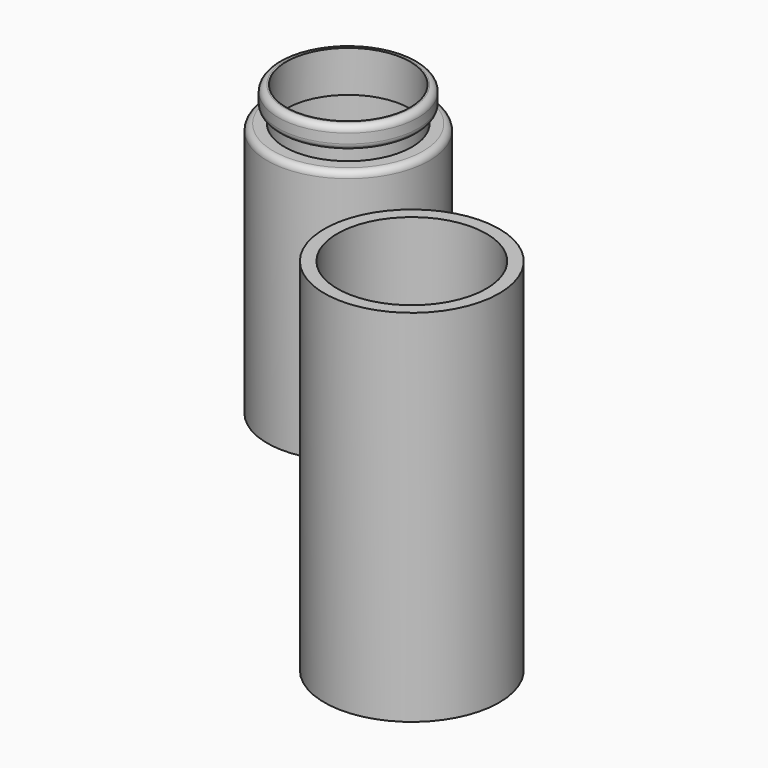
from build123d import *

# Parameters (mm, degrees)
F0_R          = 13.75
F0_R_2        = 11.72
F1_DEPTH      = 2
F2_DEPTH      = 56.64
F3_R          = 12.75
F3_R_2        = 12.25
F4_DEPTH      = 38
F4_DEPTH_BACK = 1
F5_DEPTH      = 1
F6_R          = 12.75
F6_R_2        = 10
F6_R_3        = 9.75
F7_DEPTH      = 1.1
F8_DEPTH      = 3
F9_R          = 11
F9_R_2        = 10
F9_R_3        = 9.75
F10_DEPTH     = 3.5
F11_R         = 1
F12_R         = 0.99999


# Not quite as in the source:
# - a fillet or chamfer is up to 0.001 mm smaller than in the source, because OpenCascade refuses the exact size


with BuildPart() as f1:
    # F0 (on Top) → F1 (new body)
    with BuildSketch(Plane.XY):
        Circle(F0_R)
        Circle(F0_R_2, mode=Mode.SUBTRACT)
        Circle(F0_R_2)
    extrude(amount=F1_DEPTH)

    # F0 (on Top) → F2 (join)
    with BuildSketch(Plane.XY):
        Circle(F0_R)
        Circle(F0_R_2, mode=Mode.SUBTRACT)
    extrude(amount=F2_DEPTH)


with BuildPart() as f4:
    # F3 (on Top) → F4 (new body, two sides)
    with BuildSketch(Plane.XY) as f4_sk:
        with Locations((-50, 50)):
            Circle(F3_R)
        with Locations((-50, 50)):
            Circle(F3_R_2, mode=Mode.SUBTRACT)
    extrude(amount=F4_DEPTH)
    extrude(f4_sk.sketch, amount=-F4_DEPTH_BACK)

    # F3 (on Top) → F5 (join)
    with BuildSketch(Plane.XY):
        with Locations((-50, 50)):
            Circle(F3_R_2)
    extrude(amount=-F5_DEPTH)

    # F6 (on face) → F7 (join)
    with BuildSketch(Plane.XY.offset(38)):
        with Locations((-50, 50)):
            Circle(F6_R)
        with Locations((-50, 50)):
            Circle(F6_R_2, mode=Mode.SUBTRACT)
        with Locations((-50, 50)):
            Circle(F6_R_2)
        with Locations((-50, 50)):
            Circle(F6_R_3, mode=Mode.SUBTRACT)
    extrude(amount=F7_DEPTH)

    # F6 (on face) → F8 (join)
    with BuildSketch(Plane.XY.offset(38)):
        with Locations((-50, 50)):
            Circle(F6_R_2)
        with Locations((-50, 50)):
            Circle(F6_R_3, mode=Mode.SUBTRACT)
    extrude(amount=F8_DEPTH)

    # F9 (on face) → F10 (join)
    with BuildSketch(Plane.XY.offset(41)):
        with Locations((-50, 50)):
            Circle(F9_R)
        with Locations((-50, 50)):
            Circle(F9_R_2, mode=Mode.SUBTRACT)
        with Locations((-50, 50)):
            Circle(F9_R_2)
        with Locations((-50, 50)):
            Circle(F9_R_3, mode=Mode.SUBTRACT)
    extrude(amount=F10_DEPTH)

    # F11
    f11_edges = [f4.edges().sort_by_distance(p)[0] for p in [
        (-62.75, 50, 39.1),
    ]]
    fillet(f11_edges, radius=F11_R)

    # F12 (radius 1 in the source; OpenCascade refuses exactly that, so slightly less here)
    f12_edges = [f4.edges().sort_by_distance(p)[0] for p in [
        (-61, 50, 41),
        (-61, 50, 44.5),
    ]]
    fillet(f12_edges, radius=F12_R)


solid = Compound([f1.part, f4.part])
